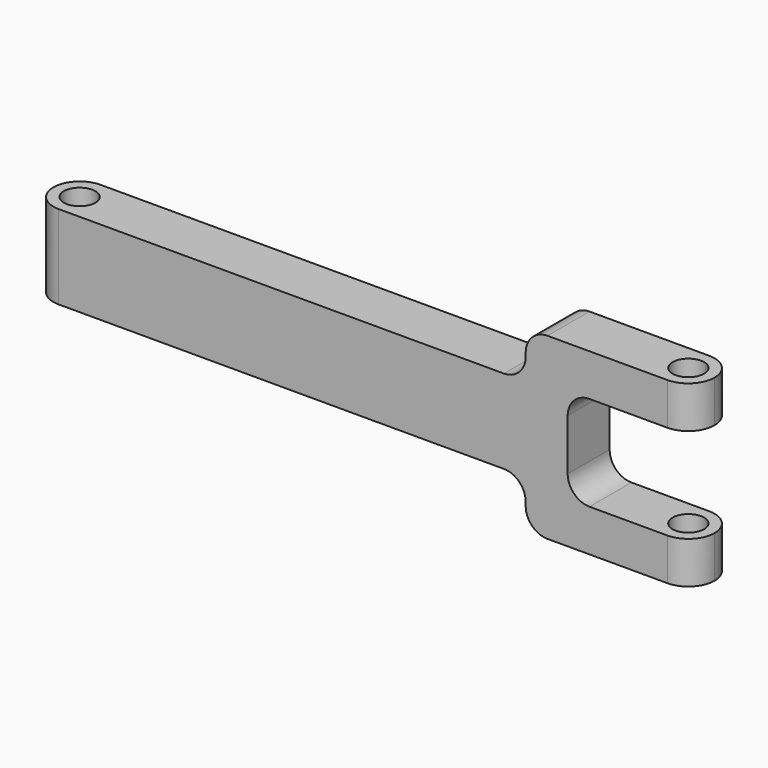
from build123d import *

# Parameters (mm, degrees)
F1_DEPTH = 54.102
F2_D     = 9.525
F3_W     = 25.4
F3_H     = 28.702
F3_W_2   = 38.1
F4_DEPTH = 25.4
F5_R     = 6.604
F6_W     = 141.2875
F6_H     = 14.351
F6_W_2   = 7.9375
F7_DEPTH = 25.4
F9_R     = 6.604


# Not quite as in the source:
# - a pattern or mirror of a feature is missing from the dataset's text; its kind, count and spacing are read off the source's solid


with BuildPart() as f1:
    # F0 (on Top) → F1 (new body)
    with BuildSketch(Plane.XY):
        with BuildLine():
            ThreePointArc((192.0875, -7.9375), (189.7626600757, -2.3248399243), (184.15, 0))
            Line((184.15, 0), (184.15, -15.875))
            ThreePointArc((184.15, -15.875), (189.7626600757, -13.5501600757), (192.0875, -7.9375))
        make_face()
        with BuildLine():
            Line((184.15, -15.875), (184.15, 0))
            ThreePointArc((184.15, 0), (176.2125, -7.9375), (184.15, -15.875))
        make_face()
        with BuildLine():
            Line((184.15, 0), (0, 0))
            ThreePointArc((0, 0), (5.6126600757, -2.3248399243), (7.9375, -7.9375))
            ThreePointArc((7.9375, -7.9375), (5.6126600757, -13.5501600757), (0, -15.875))
            Line((0, -15.875), (184.15, -15.875))
            ThreePointArc((184.15, -15.875), (176.2125, -7.9375), (184.15, 0))
        make_face()
        with BuildLine():
            ThreePointArc((7.9375, -7.9375), (5.6126600757, -2.3248399243), (0, 0))
            Line((0, 0), (0, -15.875))
            ThreePointArc((0, -15.875), (5.6126600757, -13.5501600757), (7.9375, -7.9375))
        make_face()
        with BuildLine():
            Line((0, -15.875), (0, 0))
            ThreePointArc((0, 0), (-7.9375, -7.9375), (0, -15.875))
        make_face()
    extrude(amount=F1_DEPTH)

    # F2 (through all)
    with Locations(Plane(origin=(0, 0, 0), x_dir=(1, 0, 0), z_dir=(0, 0, -1))):
        with Locations((0, 7.9375), (184.15, 7.9375)):
            Hole(F2_D / 2)

    # F3 (on Front) → F4 (cut)
    with BuildSketch(Plane.XZ):
        with Locations((204.7875, 27.051)):
            Rectangle(F3_W, F3_H)
        with Locations((173.0375, 27.051)):
            Rectangle(F3_W_2, F3_H)
    extrude(amount=F4_DEPTH, mode=Mode.SUBTRACT)

    # F5
    f5_edges = [f1.edges().sort_by_distance(p)[0] for p in [
        (153.9875, -7.9375, 41.402),
        (153.9875, -7.9375, 12.7),
    ]]
    fillet(f5_edges, radius=F5_R)

    # F6 (on Front) → F7 (cut)
    with BuildSketch(Plane.XZ):
        with Locations((70.64375, 46.9265)):
            Rectangle(F6_W, F6_H)
        with Locations((-3.96875, 46.9265)):
            Rectangle(F6_W_2, F6_H)
        Polygon((-20.6375, 39.751), (-7.9375, 39.751), (-7.9375, 54.102), (0, 54.102), (141.2875, 54.102), (141.2875, 66.802), (-20.6375, 66.802), align=None)
    f7 = extrude(amount=F7_DEPTH, mode=Mode.SUBTRACT)

    # F7_copies: F7 across plane
    add(f7.mirror(Plane(origin=(0, 0, 27.051), x_dir=(-1, 0, 0), z_dir=(0, 0, -1))), mode=Mode.SUBTRACT)

    # F9
    f9_edges = [f1.edges().sort_by_distance(p)[0] for p in [
        (141.2875, -7.9375, 39.751),
        (141.2875, -7.9375, 54.102),
        (141.2875, -7.9375, 0),
        (141.2875, -7.9375, 14.351),
    ]]
    fillet(f9_edges, radius=F9_R)


solid = f1.part
